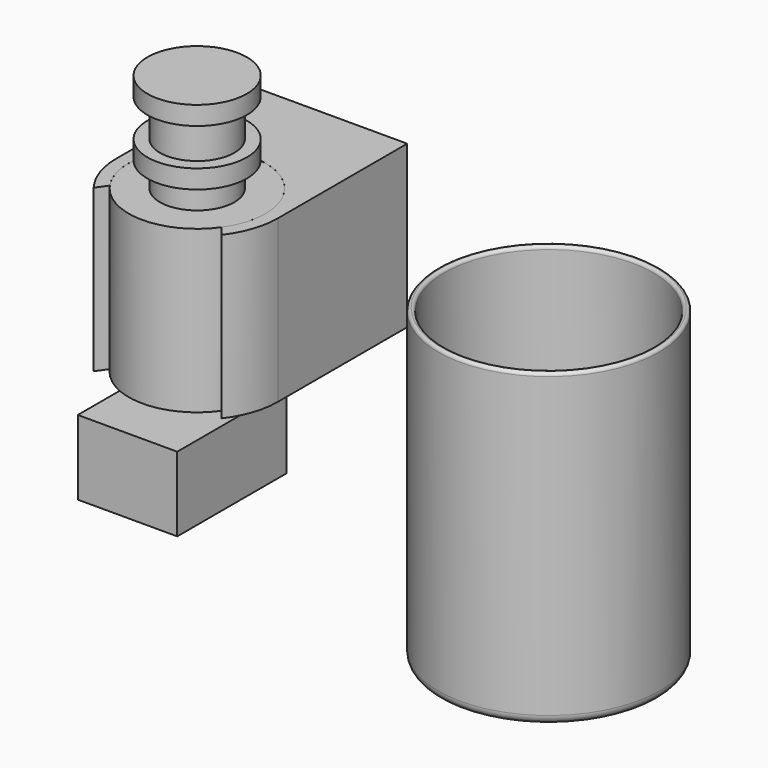
from build123d import *

# Parameters (mm, degrees)
F2_W     = 16
F2_H     = 22
F2_R     = 4
F2_R_2   = 2.5
F3_DEPTH = 12
F5_DEPTH = 26
F6_W     = 15
F6_H     = 1
F8_R     = 1.5
F9_R     = 0.49999
F9_2_R   = 0.49999


# Not quite as in the source:
# - a fillet or chamfer is up to 0.001 mm smaller than in the source, because OpenCascade refuses the exact size


with BuildPart() as f1:
    # F0 (on Front) → F1 (revolve)
    with BuildSketch(Plane.XZ):
        Polygon((8, 62.5), (0, 62.5), (0, 0), (4, 3), (4, 5.5), (2.5, 5.5), (2.5, 20.5), (11, 20.5), (11, 46.5), (6, 46.5), (6, 50.5), (8, 50.5), (8, 53.5), (6, 53.5), (6, 59.5), (8, 59.5), align=None)
    revolve(axis=Axis((0, 0, 31.25), (0, 0, 1)))

    # F2 (on face) → F3 (join)
    with BuildSketch(Plane.XY.offset(5.5)):
        with Locations((0, -3)):
            Rectangle(F2_W, F2_H)
        Circle(F2_R, mode=Mode.SUBTRACT)
        Circle(F2_R)
        Circle(F2_R_2, mode=Mode.SUBTRACT)
        Circle(F2_R_2)
    extrude(amount=F3_DEPTH)


with BuildPart() as f5:
    # F4 (on face) → F5 (new body)
    with BuildSketch(Plane.XY.offset(46.5)):
        with BuildLine():
            Line((8.9825857509, -6.349263991), (10.2716757383, -7.9682292592))
            ThreePointArc((10.2716757383, -7.9682292592), (12.2990199731, -4.2111883953), (13, 0))
            Line((13, 0), (13, 26))
            Line((13, 26), (-13, 26))
            Line((-13, 26), (-13, 0))
            ThreePointArc((-13, 0), (-12.2990199731, -4.2111883953), (-10.2716757383, -7.9682292592))
            Line((-10.2716757383, -7.9682292592), (-9.0506829178, -6.2518108354))
            ThreePointArc((-9.0506829178, -6.2518108354), (-3.2743310694, 10.5013692463), (11, 0))
            ThreePointArc((11, 0), (10.4835214327, -3.3310326282), (8.9825857509, -6.349263991))
        make_face()
    extrude(amount=-F5_DEPTH)


with BuildPart() as f7:
    # F6 (on Front) → F7 (revolve)
    with BuildSketch(Plane.XZ):
        Polygon((73.3825470388, -1), (70.0825470388, -1), (70.0825470388, -2), (74.3825470388, -2), (74.3825470388, 48), (73.3825470388, 48), align=None)
    revolve(axis=Axis((56.5825470388, 0, 14.3292332895), (0, 0, -1)))

    # F8
    f8_edges = [f7.edges().sort_by_distance(p)[0] for p in [
        (38.782547, 0, -2),
    ]]
    fillet(f8_edges, radius=F8_R)

    # F9 (radius 0.5 in the source; OpenCascade refuses exactly that, so slightly less here)
    f9_edges = [f7.edges().sort_by_distance(p)[0] for p in [
        (39.782547, 0, -1),
        (43.082547, 0, -1),
        (43.082547, 0, -2),
        (38.782547, 0, 48),
        (39.782547, 0, 48),
    ]]
    fillet(f9_edges, radius=F9_R)


with BuildPart() as f7b:
    # F6 (on Front) → F7, piece 2 (revolve)
    with BuildSketch(Plane.XZ):
        with Locations((65.5825470388, 0.5)):
            Rectangle(F6_W, F6_H)
    revolve(axis=Axis((56.5825470388, 0, 14.3292332895), (0, 0, -1)))

    # F9#2 (radius 0.5 in the source; OpenCascade refuses exactly that, so slightly less here)
    f9_2_edges = [f7b.edges().sort_by_distance(p)[0] for p in [
        (40.082547, 0, 1),
        (55.082547, 0, 1),
        (40.082547, 0, 0),
        (55.082547, 0, 0),
    ]]
    fillet(f9_2_edges, radius=F9_2_R)


solid = Compound([f1.part, f5.part, f7.part, f7b.part])
